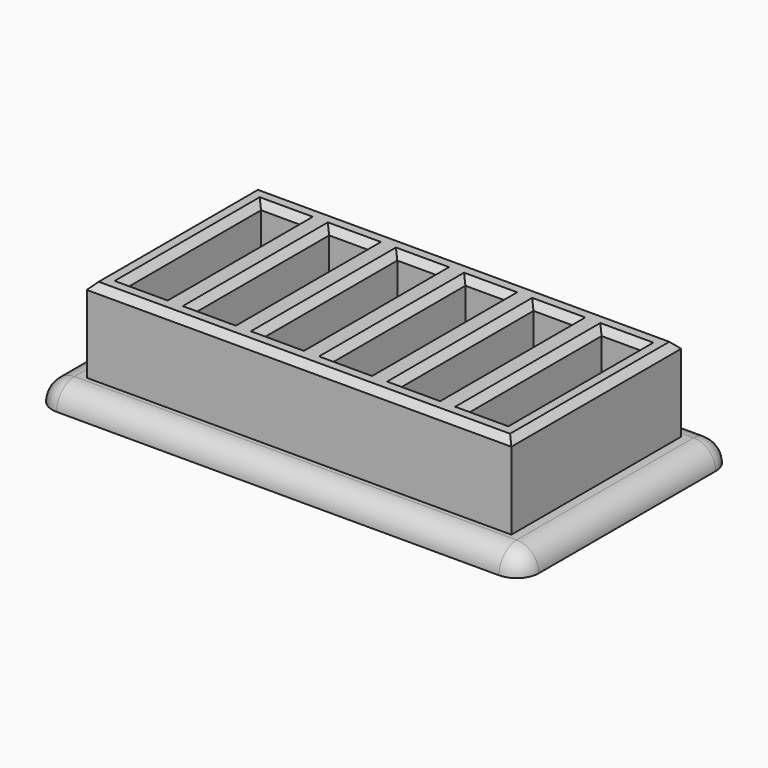
from build123d import *

# Parameters (mm, degrees)
F0_W     = 96
F0_H     = 48
F1_DEPTH = 2
F2_W     = 96
F2_H     = 48
F2_W_2   = 9
F2_H_2   = 38
F3_DEPTH = 22
F0_W_2   = 110
F0_H_2   = 60
F4_DEPTH = 5
F5_R     = 4.99999
F6_SIZE  = 1.5


# Not quite as in the source:
# - a fillet or chamfer is up to 0.001 mm smaller than in the source, because OpenCascade refuses the exact size
# - a feature names something its author has since deleted; it is built from what else it names


with BuildPart() as f1:
    # F0 (on Top) → F1 (new body)
    with BuildSketch(Plane.XY):
        Rectangle(F0_W, F0_H)
    extrude(amount=F1_DEPTH)

    # F2 (on face) → F3 (join)
    with BuildSketch(Plane.XY.offset(2)):
        Rectangle(F2_W, F2_H)
        with Locations((-38.5, 0)):
            Rectangle(F2_W_2, F2_H_2, mode=Mode.SUBTRACT)
        with Locations((-23.1, 0)):
            Rectangle(F2_W_2, F2_H_2, mode=Mode.SUBTRACT)
        with Locations((-7.7, 0)):
            Rectangle(F2_W_2, F2_H_2, mode=Mode.SUBTRACT)
        with Locations((7.7, 0)):
            Rectangle(F2_W_2, F2_H_2, mode=Mode.SUBTRACT)
        with Locations((23.1, 0)):
            Rectangle(F2_W_2, F2_H_2, mode=Mode.SUBTRACT)
        with Locations((38.5, 0)):
            Rectangle(F2_W_2, F2_H_2, mode=Mode.SUBTRACT)
    extrude(amount=F3_DEPTH)

    # F0 (on Top) → F4 (join)
    with BuildSketch(Plane.XY):
        Rectangle(F0_W_2, F0_H_2)
        Rectangle(F0_W, F0_H, mode=Mode.SUBTRACT)
    extrude(amount=F4_DEPTH)

    # F5 (radius 5 in the source; OpenCascade refuses exactly that, so slightly less here)
    f5_edges = [f1.edges().sort_by_distance(p)[0] for p in [
        (0, -30, 5),
        (-55, 0, 5),
        (0, 30, 5),
        (55, 0, 5),
        (55, -30, 2.5),
        (55, 30, 2.5),
        (-55, -30, 2.5),
        (-55, 30, 2.5),
    ]]
    fillet(f5_edges, radius=F5_R)

    # F6
    f6_edges = [f1.edges().sort_by_distance(p)[0] for p in [
        (0, -24, 24),
        (-48, 0, 24),
        (0, 24, 24),
        (48, 0, 24),
        (-43, 0, 24),
        (-34, 0, 24),
        (-38.5, -19, 24),
        (-38.5, 19, 24),
        (-23.1, -19, 24),
        (-18.6, 0, 24),
        (-27.6, 0, 24),
        (-23.1, 19, 24),
        (-7.7, 19, 24),
        (-12.2, 0, 24),
        (-7.7, -19, 24),
        (-3.2, 0, 24),
        (3.2, 0, 24),
        (12.2, 0, 24),
        (7.7, -19, 24),
        (7.7, 19, 24),
        (18.6, 0, 24),
        (23.1, 19, 24),
        (27.6, 0, 24),
        (23.1, -19, 24),
        (38.5, -19, 24),
        (34, 0, 24),
        (43, 0, 24),
        (38.5, 19, 24),
    ]]
    chamfer(f6_edges, length=F6_SIZE)


solid = f1.part
